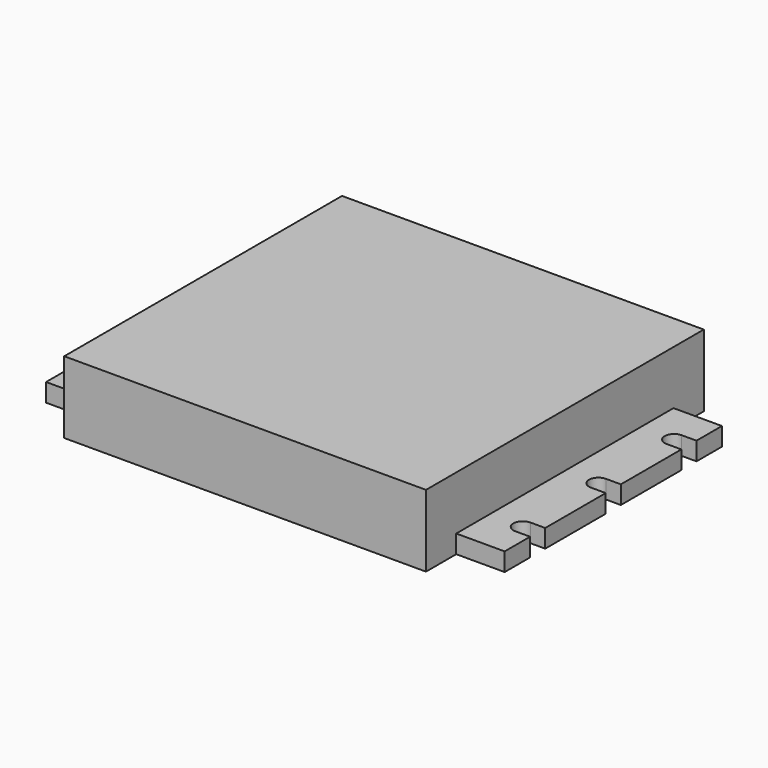
from build123d import *

# Parameters (mm, degrees)
F0_W     = 63.14
F0_H     = 60.6
F1_DEPTH = 12.57
F2_W     = 47.4
F2_H     = 3.18
F3_DEPTH = 8.45
F5_W     = 2.59
F5_H     = 3.3
F6_DEPTH = 3.18


# Not quite as in the source:
# - a feature names something its author has since deleted; it is built from what else it names


with BuildPart() as f1:
    # F0 (on Top) → F1 (new body)
    with BuildSketch(Plane.XY):
        Rectangle(F0_W, F0_H)
    extrude(amount=F1_DEPTH)

    # F2 (on face) → F3 (join)
    with BuildSketch(Plane(origin=(-31.57, 0, 0), x_dir=(0, -1, 0), z_dir=(-1, 0, 0))):
        with Locations((0, 1.59)):
            Rectangle(F2_W, F2_H)
    extrude(amount=F3_DEPTH)

    # F4: F1 across plane


with BuildPart() as f1_1:
    add(f1.part)
    add(f1.part.mirror(Plane.YZ))

    # F5 (on face) → F6 (cut, through all)
    with BuildSketch(Plane.XY.offset(3.18)):
        with Locations((-38.725, 16.5)):
            Rectangle(F5_W, F5_H)
        with BuildLine():
            Line((-37.43, 18.15), (-37.43, 14.85))
            ThreePointArc((-37.43, 14.85), (-35.78, 16.5), (-37.43, 18.15))
        make_face()
        with Locations((-38.725, 0)):
            Rectangle(F5_W, F5_H)
        with BuildLine():
            ThreePointArc((-37.43, -1.65), (-35.78, 0), (-37.43, 1.65))
            Line((-37.43, 1.65), (-37.43, -1.65))
        make_face()
        with Locations((-38.725, -16.5)):
            Rectangle(F5_W, F5_H)
        with BuildLine():
            ThreePointArc((-37.43, -18.15), (-35.78, -16.5), (-37.43, -14.85))
            Line((-37.43, -14.85), (-37.43, -18.15))
        make_face()
        with BuildLine():
            Line((37.43, 14.85), (37.43, 18.15))
            ThreePointArc((37.43, 18.15), (35.78, 16.5), (37.43, 14.85))
        make_face()
        with Locations((38.725, 16.5)):
            Rectangle(F5_W, F5_H)
        with BuildLine():
            ThreePointArc((37.43, 1.65), (35.78, 0), (37.43, -1.65))
            Line((37.43, -1.65), (37.43, 1.65))
        make_face()
        with Locations((38.725, 0)):
            Rectangle(F5_W, F5_H)
        with BuildLine():
            ThreePointArc((37.43, -14.85), (35.78, -16.5), (37.43, -18.15))
            Line((37.43, -18.15), (37.43, -14.85))
        make_face()
        with Locations((38.725, -16.5)):
            Rectangle(F5_W, F5_H)
    extrude(amount=-F6_DEPTH, mode=Mode.SUBTRACT)


solid = f1_1.part
